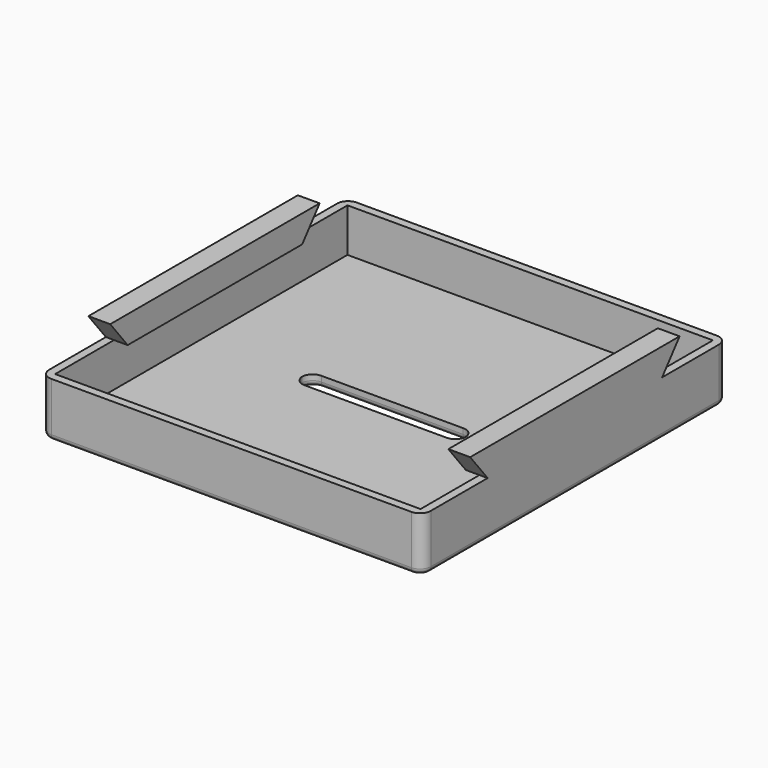
from build123d import *

# Parameters (mm, degrees)
F0_W        = 177.8
F0_H        = 177.8
F0_W_2      = 170.18
F0_H_2      = 170.18
F1_DEPTH    = 25.4
F0_W_3      = 76.2
F0_H_3      = 9.652
F2_DEPTH    = 5.08
F3_T1_DEPTH = 5.08
F5_DEPTH    = 177.8
F6_W        = 78.74
F6_H        = 15.522254324
F7_DEPTH    = 177.801
F8_R        = 5.08
F9_R        = 2.54


# Not quite as in the source:
# - a fillet or chamfer that OpenCascade refuses, or shapes differently, is made with other operations: its cross-section is extruded or revolved along the edge and cut away or added


with BuildPart() as f1:
    # F0 (on Top) → F1 (new body)
    with BuildSketch(Plane.XY):
        Rectangle(F0_W, F0_H)
        Rectangle(F0_W_2, F0_H_2, mode=Mode.SUBTRACT)
    extrude(amount=F1_DEPTH)

    # F0 (on Top) → F2 (join)
    with BuildSketch(Plane.XY):
        Rectangle(F0_W_2, F0_H_2)
        Rectangle(F0_W_3, F0_H_3, mode=Mode.SUBTRACT)
    extrude(amount=F2_DEPTH)

    # F3: fillet of radius 5.08 on 4 edges, made by hand

    # F3_s2 → F3_t1 (join)
    with BuildSketch(Plane.XY):
        with BuildLine():
            ThreePointArc((33.02, 4.826), (36.6121024484, 3.3381024484), (38.1, -0.254))
            Line((38.1, -0.254), (38.1, 4.826))
            Line((38.1, 4.826), (33.02, 4.826))
        make_face()
        with BuildLine():
            ThreePointArc((38.1, 0.254), (36.6121024484, -3.3381024484), (33.02, -4.826))
            Line((33.02, -4.826), (38.1, -4.826))
            Line((38.1, -4.826), (38.1, 0.254))
        make_face()
        with BuildLine():
            ThreePointArc((-38.1, -0.254), (-36.6121024484, 3.3381024484), (-33.02, 4.826))
            Line((-33.02, 4.826), (-38.1, 4.826))
            Line((-38.1, 4.826), (-38.1, -0.254))
        make_face()
        with BuildLine():
            ThreePointArc((-38.1, 0.254), (-36.6121024484, -3.3381024484), (-33.02, -4.826))
            Line((-33.02, -4.826), (-38.1, -4.826))
            Line((-38.1, -4.826), (-38.1, 0.254))
        make_face()
    extrude(amount=F3_T1_DEPTH)

    # F4 (on face) → F5 (join, through all)
    with BuildSketch(Plane.YZ.offset(88.9)):
        Polygon((-50.8, 25.4), (0, 25.4), (0, 38.1), (-60.96, 38.1), align=None)
        Polygon((0, 38.1), (0, 25.4), (50.8, 25.4), (60.96, 38.1), align=None)
    extrude(amount=-F5_DEPTH)

    # F6 (on face) → F7 (cut, through all)
    with BuildSketch(Plane(origin=(0, 88.9, 0), x_dir=(-1, 0, 0), z_dir=(0, 1, 0))):
        with Locations((-39.37, 33.161127162)):
            Rectangle(F6_W, F6_H)
        with Locations((39.37, 33.161127162)):
            Rectangle(F6_W, F6_H)
    extrude(amount=-F7_DEPTH, mode=Mode.SUBTRACT)

    # F8
    f8_edges = [f1.edges().sort_by_distance(p)[0] for p in [
        (88.9, -88.9, 12.7),
        (88.9, 88.9, 12.7),
        (-88.9, 88.9, 12.7),
        (-88.9, -88.9, 12.7),
    ]]
    fillet(f8_edges, radius=F8_R)

    # F9
    f9_edges = [f1.edges().sort_by_distance(p)[0] for p in [
        (88.9, 0, 0),
        (0, 88.9, 0),
        (87.412102, -87.412102, 0),
        (87.412102, 87.412102, 0),
        (0, -88.9, 0),
        (-87.412102, -87.412102, 0),
        (-87.412102, 87.412102, 0),
        (-88.9, 0, 0),
        (0, -4.826, 0),
        (-36.521148, -3.42681, 0),
        (-36.521148, 3.42681, 0),
        (0, 4.826, 0),
        (36.521148, 3.42681, 0),
        (36.521148, -3.42681, 0),
    ]]
    fillet(f9_edges, radius=F9_R)


solid = f1.part
